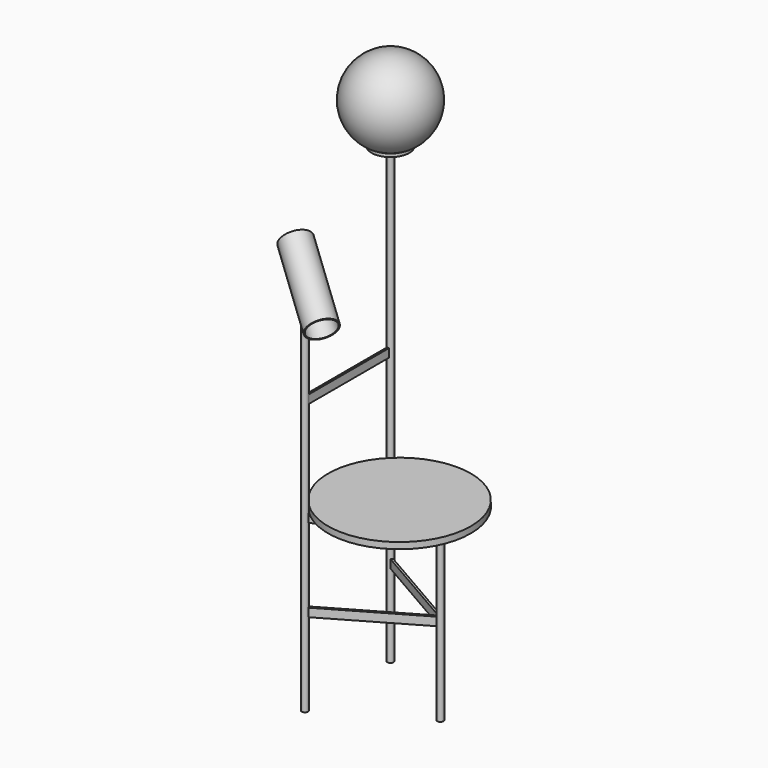
from build123d import *

# Parameters (mm, degrees)
F1_R           = 9.525
F1_R_2         = 6.35
F2_DEPTH       = 1371.6
F3_R           = 9.525
F3_R_2         = 6.35
F4_DEPTH       = 1079.5
F5_R           = 9.525
F5_R_2         = 6.35
F6_DEPTH       = 527.05
F10_R          = 215.9
F11_DEPTH      = 19.05
F17_ANGLE      = 125
F23_W          = 6.35
F23_H          = 25.4
F24_DEPTH      = 153.9447438789
F24_DEPTH_BACK = 153.9447438789
F25_W          = 6.35
F25_H          = 25.4
F26_DEPTH      = 153.9447438789
F26_DEPTH_BACK = 153.9447438789
F28_DEPTH      = 3.175
F29_W          = 6.35
F29_H          = 25.4
F30_REACH      = 477.0327207227
F32_W          = 57.15
F32_H          = 9.525
F37_REACH      = 477.0327207227
F42_R          = 4.365625
F43_DEPTH      = 25.4
F45_R          = 4.365625
F46_REACH      = 525.921615725
F47_R          = 4.365625
F48_DEPTH      = 3.175
F52_ANGLE      = 35
F53_R          = 7.9375
F54_DEPTH      = 19.05


# Not quite as in the source:
# - a feature of the source that left no trace in its solid (it failed there, or was rolled back) is left out
# - a feature names something its author has since deleted; it is built from what else it names


with BuildPart() as f2:
    # F1 (on Top) → F2 (new body)
    with BuildSketch(Plane.XY):
        with Locations((0, 161.925)):
            Circle(F1_R)
        with Locations((0, 161.925)):
            Circle(F1_R_2, mode=Mode.SUBTRACT)
    extrude(amount=F2_DEPTH)



with BuildPart() as f4:
    # F3 (on Top) → F4 (new body)
    with BuildSketch(Plane.XY):
        with Locations((0, -161.925)):
            Circle(F3_R)
        with Locations((0, -161.925)):
            Circle(F3_R_2, mode=Mode.SUBTRACT)
    extrude(amount=F4_DEPTH)



with BuildPart() as f6:
    # F5 (on Top) → F6 (new body)
    with BuildSketch(Plane.XY):
        with Locations((280.4623270156, 0)):
            Circle(F5_R)
        with Locations((280.4623270156, 0)):
            Circle(F5_R_2, mode=Mode.SUBTRACT)
    extrude(amount=F6_DEPTH)


with BuildPart() as f9:
    # F8 (on offset) → F9 (revolve)
    with BuildSketch(Plane.XY.offset(1473.2)):
        with BuildLine():
            Line((-127, 161.925), (127, 161.925))
            ThreePointArc((127, 161.925), (0, 288.925), (-127, 161.925))
        make_face()
    revolve(axis=Axis((0, 161.925, 1473.2), (1, 0, 0)))


with BuildPart() as f11:
    # F10 (on face) → F11 (new body)
    with BuildSketch(Plane.XY.offset(527.05)):
        with Locations((156.8334307474, 0)):
            Circle(F10_R)
    extrude(amount=F11_DEPTH)


with BuildPart() as f14:
    # F13 (on Right) → F14 (revolve)
    with BuildSketch(Plane.YZ):
        Polygon((-251.7275612107, 1169.3025612107), (-72.1224387893, 989.6974387893), (-40.6915423656, 1021.1283352131), (-220.2966647869, 1200.7334576344), align=None)
    revolve(axis=Axis((0, -130.4941035763, 1110.9308964237), (0, 0.7071067812, -0.7071067812)))


with BuildPart() as f14_1:
    # F17: moved
    add(f14.part.rotate(Axis((0, -161.925, -47.2708940506), (0, 0, -1)), F17_ANGLE))


with BuildPart() as f4_1:
    add(f4.part)

    add(f6.part)  # F24 merges F6
    # F23 (on line) → F24 (join, two sides)
    with BuildSketch(Plane(origin=(70.1155817539, 40.48125, 0), x_dir=(0.5, -0.8660254038, 0), z_dir=(-0.8660254038, -0.5, 0))) as f24_sk:
        with Locations((140.2311635078, 263.525)):
            Rectangle(F23_W, F23_H)
        with Locations((140.2311635078, 514.35)):
            Rectangle(F23_W, F23_H)
    extrude(amount=F24_DEPTH)
    extrude(f24_sk.sketch, amount=-F24_DEPTH_BACK)


with BuildPart() as f2_1:
    add(f2.part)

    add(f4_1.part)  # F26 merges F4
    # F25 (on line) → F26 (join, two sides)
    with BuildSketch(Plane(origin=(70.1155817539, -40.48125, 0), x_dir=(0.5, 0.8660254038, 0), z_dir=(0.8660254038, -0.5, 0))) as f26_sk:
        with Locations((140.2311635078, 263.525)):
            Rectangle(F25_W, F25_H)
        with Locations((140.2311635078, 514.35)):
            Rectangle(F25_W, F25_H)
    extrude(amount=F26_DEPTH)
    extrude(f26_sk.sketch, amount=-F26_DEPTH_BACK)

    f30_end = f2_1.faces().sort_by_distance((-9.525, 161.925, 685.8))[0]
    # F29 (on plane+point) → F30 (join, up to a face of the model that its end follows)
    with BuildSketch(Plane.XZ.offset(161.925)):
        with Locations((0, 514.35)):
            Rectangle(F29_W, F29_H)
    f30_long = extrude(amount=-F30_REACH, mode=Mode.PRIVATE)
    add(split(f30_long, bisect_by=f30_end, keep=Keep.ALL, mode=Mode.PRIVATE).solids().sort_by_distance((0, -161.925, 514.35))[0])

    f37_end = f2_1.faces().sort_by_distance((-9.525, 161.925, 685.8))[0]
    # F36 (on plane+point) → F37 (join, up to a face of the model that its end follows)
    with BuildSketch(Plane.XZ.offset(161.925)):
        Polygon((3.175, 812.8), (3.175, 838.2), (-3.175, 838.2), (-3.175, 812.8), (0, 812.8), align=None)
    f37_long = extrude(amount=-F37_REACH, mode=Mode.PRIVATE)
    add(split(f37_long, bisect_by=f37_end, keep=Keep.ALL, mode=Mode.PRIVATE).solids().sort_by_distance((0, -161.925, 825.5))[0])

    # F41: union 

    # F42 (on Right) → F43 (cut)
    with BuildSketch(Plane.YZ):
        with Locations((161.925, 12.7)):
            Circle(F42_R)
    extrude(amount=-F43_DEPTH, mode=Mode.SUBTRACT)

    f46_end = f2_1.faces().sort_by_distance((-9.525, 161.925, 685.8))[0]
    # F45 (on line) → F46 (cut, up to a face of the model that its end follows)
    with BuildSketch(Plane(origin=(-70.1155817539, 121.44375, 0), x_dir=(0.8660254038, 0.5, 0), z_dir=(0.5, -0.8660254038, 0))):
        with Locations((80.9625, 492.125)):
            Circle(F45_R)
    f46_long = extrude(amount=F46_REACH, mode=Mode.PRIVATE)
    add(split(f46_long, bisect_by=f46_end, keep=Keep.BOTTOM, mode=Mode.PRIVATE), mode=Mode.SUBTRACT)


with BuildPart() as f28:
    # F27 (on face) → F28 (new body)
    with BuildSketch(Plane(origin=(0, 0, 501.65), x_dir=(1, 0, 0), z_dir=(0, 0, -1))):
        Polygon((4.7625, -153.676108029), (270.9373270156, 0), (4.7625, 153.676108029), align=None)
    extrude(amount=-F28_DEPTH)

    # F47 (on face) → F48 (cut, through all)
    with BuildSketch(Plane.XY.offset(504.825)):
        with Locations((14.2875, 137.1783240869)):
            Circle(F47_R)
    extrude(amount=-F48_DEPTH, mode=Mode.SUBTRACT)


with BuildPart() as f33:
    # F32 (on Right) → F33 (revolve)
    with BuildSketch(Plane.YZ):
        with Locations((190.5, 1376.3625)):
            Rectangle(F32_W, F32_H)
    revolve(axis=Axis((0, 161.925, 1395.9616556168), (0, 0, 1)))


with BuildPart() as f35:
    # F34 (on Right) → F35 (revolve)
    with BuildSketch(Plane.YZ):
        with BuildLine():
            Line((212.725, 1381.6149142838), (212.725, 1378.1422038299))
            ThreePointArc((212.725, 1378.1422038299), (286.2461017422, 1520.4869512303), (161.925, 1621.5396264818))
            Line((161.925, 1621.5396264818), (161.925, 1618.3646264818))
            ThreePointArc((161.925, 1618.3646264818), (282.9942634671, 1520.5177724615), (212.725, 1381.6149142838))
        make_face()
    revolve(axis=Axis((0, 161.925, 1437.8323132409), (0, 0, 1)))


with BuildPart() as f50:
    # F49 (on plane+point) → F50 (revolve)
    with BuildSketch(Plane.XZ.offset(161.925)):
        Polygon((163.9602262806, 1124.7396583964), (-56.0102262806, 1251.7396583964), (-57.5977262806, 1248.9900277394), (162.3727262806, 1121.9900277394), align=None)
    revolve(axis=Axis((31.75, -161.925, 1149.7448291982), (0.8660254038, 0, -0.5)))


with BuildPart() as f50_1:
    # F52: moved
    add(f50.part.rotate(Axis((0, -161.925, -8.3484528586), (0, 0, -1)), F52_ANGLE))


with BuildPart() as f54:
    # F53 (on face) → F54 (new body)
    with BuildSketch(Plane(origin=(-3.175, 0, 0), x_dir=(0, -1, 0), z_dir=(-1, 0, 0))):
        with Locations((4.0062814951, 514.35)):
            Circle(F53_R)
    extrude(amount=F54_DEPTH)


solid = Compound([f11.part, f2_1.part, f28.part, f33.part, f35.part, f50_1.part, f54.part])
